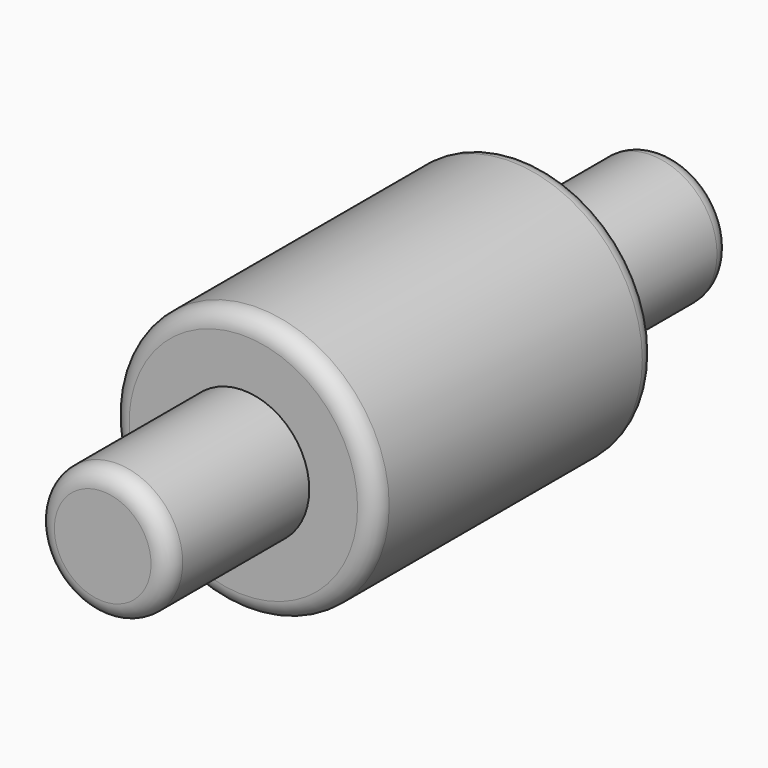
from build123d import *

# Parameters (mm, degrees)
F1_R     = 19.05
F2_DEPTH = 50.8
F0_R     = 38.1
F3_DEPTH = 101.6
F4_R     = 5.08
F5_R     = 5.08


with BuildPart() as f2:
    # F1 (on Front) → F2 (new body, symmetric)
    with BuildSketch(Plane.XZ):
        Circle(F1_R)
    extrude(amount=F2_DEPTH, both=True)


with BuildPart() as f2b:
    # F0 (on Front) → F2, piece 2 (new body, symmetric)
    with BuildSketch(Plane.XZ):
        Circle(F0_R)
    extrude(amount=F2_DEPTH, both=True)

    # F4
    f4_edges = [f2b.edges().sort_by_distance(p)[0] for p in [
        (-38.1, -50.8, 0),
        (-38.1, 50.8, 0),
    ]]
    fillet(f4_edges, radius=F4_R)


with BuildPart() as f3:
    # F1 (on Front) → F3 (new body, symmetric)
    with BuildSketch(Plane.XZ):
        Circle(F1_R)
    extrude(amount=F3_DEPTH, both=True)

    # F5
    f5_edges = [f3.edges().sort_by_distance(p)[0] for p in [
        (-19.05, 101.6, 0),
        (-19.05, -101.6, 0),
    ]]
    fillet(f5_edges, radius=F5_R)


solid = Compound([f2.part, f2b.part, f3.part])
